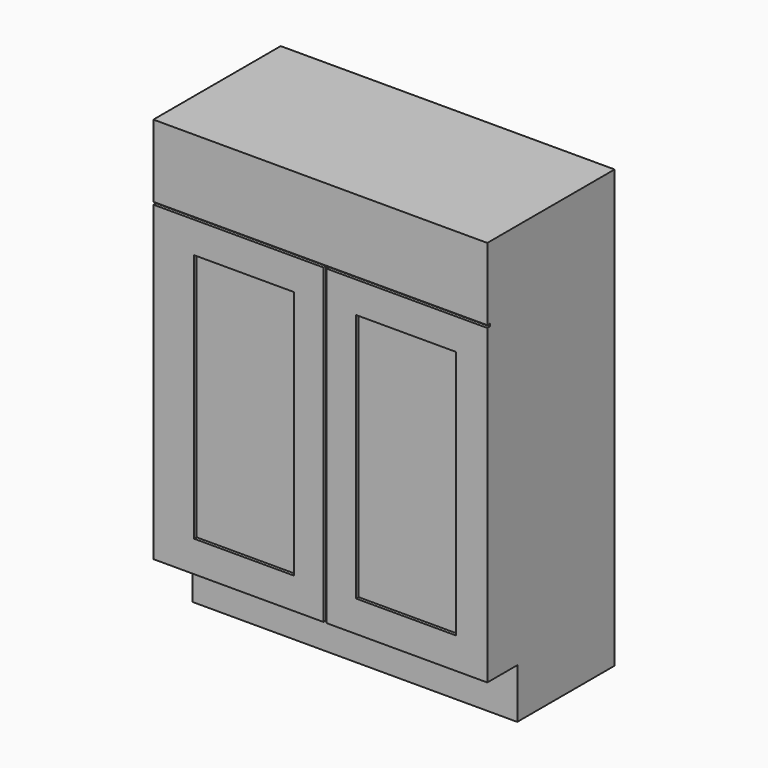
from build123d import *

# Parameters (mm, degrees)
F0_W     = 3.175
F0_H     = 635
F0_W_2   = 327.025
F0_W_3   = 203.2
F0_H_2   = 508
F0_W_4   = 330.2
F0_H_3   = 147.32
F1_DEPTH = 323.85
F2_DEPTH = 6.35
F3_DEPTH = 76.2
F4_W     = 196.85
F4_H     = 660.4
F5_DEPTH = 19.05
F6_DEPTH = 12.7


with BuildPart() as f1:
    # F0 (on Front) → F1 (new body)
    with BuildSketch(Plane.XZ):
        Polygon((0, -101.6), (0, 0), (-3.175, 0), (-330.2, 0), (-330.2, -101.6), align=None)
        with Locations((-1.5875, 317.5)):
            Rectangle(F0_W, F0_H)
        Polygon((3.175, 0), (0, 0), (0, -101.6), (330.2, -101.6), (330.2, 0), align=None)
        with Locations((1.5875, 317.5)):
            Rectangle(F0_W, F0_H)
        with Locations((-166.6875, 317.5)):
            Rectangle(F0_W_2, F0_H)
        with Locations((-165.1, 317.5)):
            Rectangle(F0_W_3, F0_H_2, mode=Mode.SUBTRACT)
        Polygon((-3.175, 635), (0, 635), (0, 640.08), (-330.2, 640.08), (-330.2, 635), align=None)
        Polygon((0, 640.08), (0, 635), (3.175, 635), (330.2, 635), (330.2, 640.08), align=None)
        with Locations((166.6875, 317.5)):
            Rectangle(F0_W_2, F0_H)
        with Locations((165.1, 317.5)):
            Rectangle(F0_W_3, F0_H_2, mode=Mode.SUBTRACT)
        with Locations((-165.1, 713.74)):
            Rectangle(F0_W_4, F0_H_3)
        with Locations((165.1, 713.74)):
            Rectangle(F0_W_4, F0_H_3)
        with Locations((-165.1, 317.5)):
            Rectangle(F0_W_3, F0_H_2)
        with Locations((165.1, 317.5)):
            Rectangle(F0_W_3, F0_H_2)
    extrude(amount=-F1_DEPTH)

    # F0 (on Front) → F2 (cut)
    with BuildSketch(Plane.XZ):
        Polygon((0, -101.6), (0, 0), (-3.175, 0), (-330.2, 0), (-330.2, -101.6), align=None)
        with Locations((-1.5875, 317.5)):
            Rectangle(F0_W, F0_H)
        with Locations((1.5875, 317.5)):
            Rectangle(F0_W, F0_H)
        Polygon((-3.175, 635), (0, 635), (0, 640.08), (-330.2, 640.08), (-330.2, 635), align=None)
        Polygon((0, 640.08), (0, 635), (3.175, 635), (330.2, 635), (330.2, 640.08), align=None)
        with Locations((-165.1, 317.5)):
            Rectangle(F0_W_3, F0_H_2)
        with Locations((165.1, 317.5)):
            Rectangle(F0_W_3, F0_H_2)
    extrude(amount=-F2_DEPTH, mode=Mode.SUBTRACT)

    # F0 (on Front) → F3 (cut)
    with BuildSketch(Plane.XZ):
        Polygon((0, -101.6), (0, 0), (-3.175, 0), (-330.2, 0), (-330.2, -101.6), align=None)
        Polygon((3.175, 0), (0, 0), (0, -101.6), (330.2, -101.6), (330.2, 0), align=None)
    extrude(amount=-F3_DEPTH, mode=Mode.SUBTRACT)

    # F4 (on face) → F5 (join)
    with BuildSketch(Plane(origin=(-330.2, 0, 0), x_dir=(0, -1, 0), z_dir=(-1, 0, 0))):
        Polygon((0, 787.4), (-323.85, 787.4), (-323.85, 0), (-76.2, 0), (0, 0), (0, 635), (-6.35, 635), (-6.35, 640.08), (0, 640.08), align=None)
        with Locations((-161.925, 393.7)):
            Rectangle(F4_W, F4_H, mode=Mode.SUBTRACT)
    extrude(amount=F5_DEPTH)

    # F6 (add): a face of the model
    f6_faces = [f1.faces().sort_by_distance(p)[0] for p in [
        (-330.2, 161.925, 393.7),
    ]]
    extrude(f6_faces, amount=F6_DEPTH)


solid = f1.part
